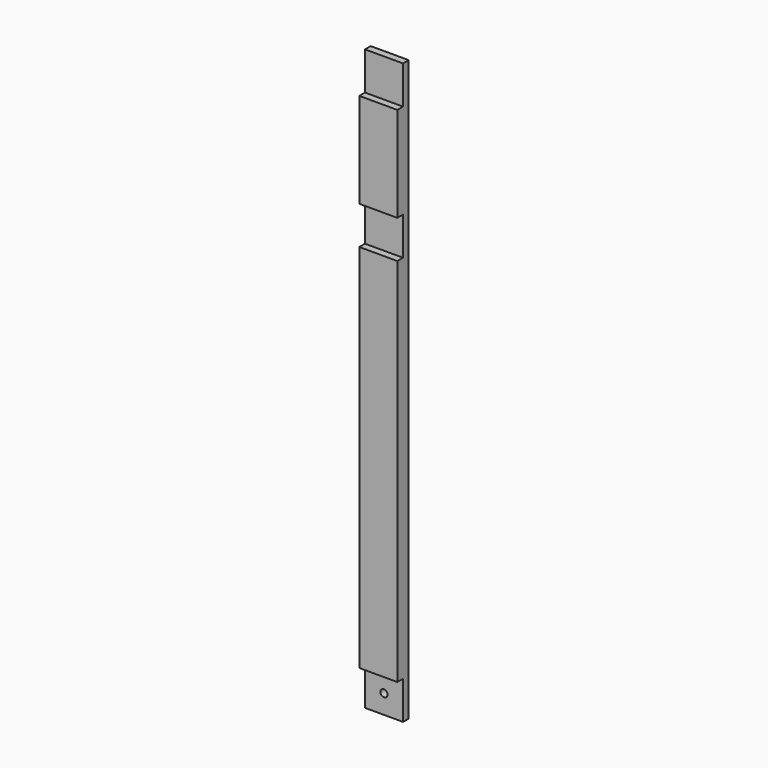
from build123d import *

# Parameters (mm, degrees)
F0_W     = 50.8
F0_H     = 19.05
F1_DEPTH = 774.7
F2_W     = 122.43557321
F2_H     = 50.8
F2_W_2   = 343.1604206562
F2_W_3   = 261.0546275973
F3_DEPTH = 25.4
F4_R     = 4.7625
F5_DEPTH = 25.4


# Not quite as in the source:
# - a feature names something its author has since deleted; it is built from what else it names


with BuildPart() as f1:
    # F0 (on Top) → F1 (new body)
    with BuildSketch(Plane.XY):
        Rectangle(F0_W, F0_H)
    extrude(amount=F1_DEPTH)

    # F2 (on Front) → F3 (cut)
    with BuildSketch(Plane.XZ):
        with Locations((22.4465244144, 25.4)):
            Rectangle(F2_W, F2_H)
        with Locations((-38.7818217278, 749.3)):
            Rectangle(F2_W_2, F2_H)
        with Locations((-37.622589618, 571.5)):
            Rectangle(F2_W_3, F2_H)
    extrude(amount=F3_DEPTH, mode=Mode.SUBTRACT)

    # F4 (on Front) → F5 (cut)
    with BuildSketch(Plane.XZ):
        with Locations((0, 25.4)):
            Circle(F4_R)
        with Locations((0, 342.9)):
            Circle(F4_R)
    extrude(amount=-F5_DEPTH, mode=Mode.SUBTRACT)


solid = f1.part
